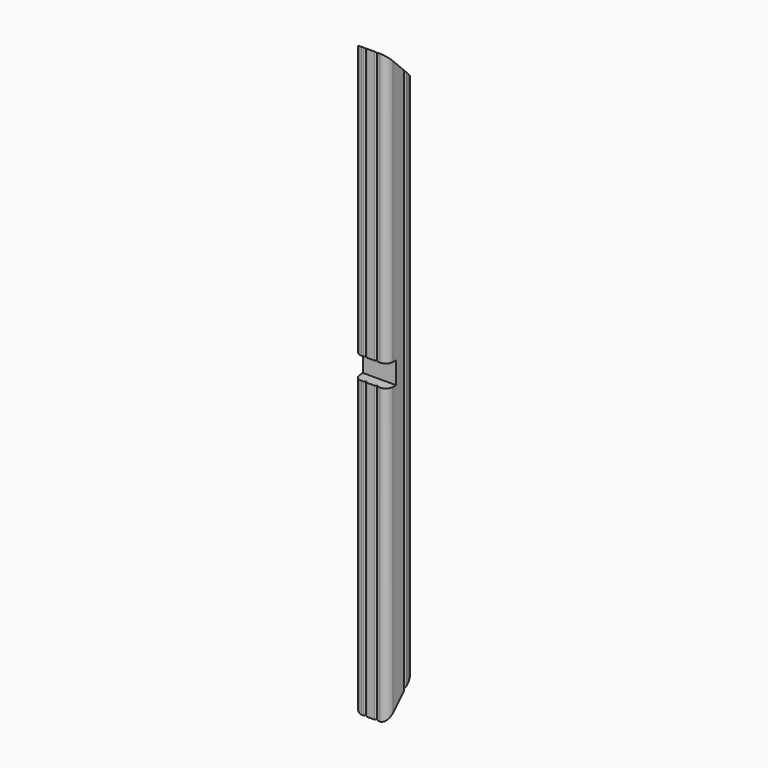
from build123d import *

# Parameters (mm, degrees)
F1_DEPTH = 1016
F3_DEPTH = 57.151
F4_W     = 19.05
F4_H     = 38.1
F5_DEPTH = 57.151


# Not quite as in the source:
# - ends of sketch curves that miss each other by under 0.0002 mm in the source are joined


with BuildPart() as f1:
    # F0 (on Top) → F1 (new body)
    with BuildSketch(Plane.XY):
        with BuildLine():
            ThreePointArc((0, 12.7), (3.7197438789, 3.7197438789), (12.7, 0))
            Line((12.7, 0), (15.9004, 0))
            ThreePointArc((15.9004, 0), (18.127503518, 0.922496482), (19.05, 3.1496))
            Line((19.05, 3.1496), (19.05, 34.9504))
            ThreePointArc((19.05, 34.9504), (18.127503518, 37.177503518), (15.9004, 38.1))
            Line((15.9004, 38.1), (3.1496, 38.1))
            ThreePointArc((3.1496, 38.1), (0.922496482, 37.177503518), (0, 34.9504))
            Line((0, 34.9504), (0, 12.7))
        make_face()
        with BuildLine():
            Line((19.05, 34.9504), (19.05, 3.1496))
            ThreePointArc((19.05, 3.1496), (19.972496482, 0.922496482), (22.1996, 0))
            Line((22.1996, 0), (34.9504, 0))
            ThreePointArc((34.9504, 0), (37.177503518, 0.922496482), (38.1, 3.1496))
            Line((38.1, 3.1496), (38.1, 34.9504))
            ThreePointArc((38.1, 34.9504), (37.177503518, 37.177503518), (34.9504, 38.1))
            Line((34.9504, 38.1), (22.1996, 38.1))
            ThreePointArc((22.1996, 38.1), (19.972496482, 37.177503518), (19.05, 34.9504))
        make_face()
        with BuildLine():
            Line((38.1, 34.9504), (38.1, 3.1496))
            ThreePointArc((38.1, 3.1496), (39.022496482, 0.922496482), (41.2496, 0))
            Line((41.2496, 0), (44.45, 0))
            ThreePointArc((44.45, 0), (53.4302561211, 3.7197438789), (57.15, 12.7))
            Line((57.15, 12.7), (57.15, 34.9504))
            ThreePointArc((57.15, 34.9504), (56.227503518, 37.177503518), (54.0004, 38.1))
            Line((54.0004, 38.1), (41.2496, 38.1))
            ThreePointArc((41.2496, 38.1), (39.022496482, 37.177503518), (38.1, 34.9504))
        make_face()
        with BuildLine():
            ThreePointArc((19.0499988437, 41.2496), (19.9724953256, 39.022496482), (22.1995988437, 38.1))
            Line((22.1995988437, 38.1), (34.9504, 38.1))
            Line((34.9504, 38.1), (41.2496, 38.1))
            Line((41.2496, 38.1), (54.0004, 38.1))
            ThreePointArc((54.0004, 38.1), (56.2275023617, 39.022496482), (57.1499988437, 41.2496))
            Line((57.1499988437, 41.2496), (57.1499988437, 44.45))
            ThreePointArc((57.1499988437, 44.45), (53.4302549647, 53.4302561211), (44.4499988437, 57.15))
            Line((44.4499988437, 57.15), (22.1995988437, 57.15))
            ThreePointArc((22.1995988437, 57.15), (19.9724953256, 56.227503518), (19.0499988437, 54.0004))
            Line((19.0499988437, 54.0004), (19.0499988437, 41.2496))
        make_face()
    extrude(amount=F1_DEPTH)

    # F2 (on face) → F3 (cut, through all)
    with BuildSketch(Plane.YZ.offset(57.15)):
        Polygon((57.15, 0), (57.15, 57.15), (0, 0), (12.7, 0), align=None)
        Polygon((12.7, 1016), (0, 1016), (57.15, 958.85), (57.15, 1016), align=None)
    extrude(amount=-F3_DEPTH, mode=Mode.SUBTRACT)

    # F4 (on face) → F5 (cut, through all)
    with BuildSketch(Plane.YZ.offset(57.15)):
        with Locations((9.525, 527.05)):
            Rectangle(F4_W, F4_H)
    extrude(amount=-F5_DEPTH, mode=Mode.SUBTRACT)


solid = f1.part
